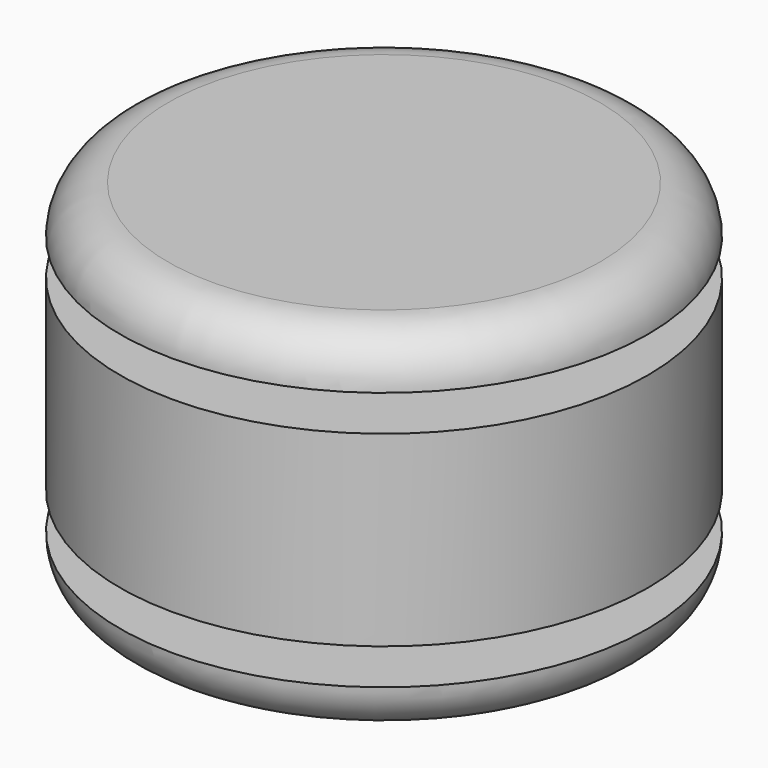
from build123d import *
from build123d import SkipClean  # not in build123d's __all__

# Parameters (mm, degrees)
F0_R      = 5.4
F1_DEPTH  = 1.5
F2_R      = 8.4
F2_R_2    = 6.4
F3_DEPTH  = 4.8
F4_R      = 11
F4_R_2    = 8.5
F5_DEPTH  = 7.8
F6_R      = 11
F6_R_2    = 5.4
F7_DEPTH  = 1.5
F8_R      = 3.15
F9_DEPTH  = 4.8
F10_R     = 4.15
F11_DEPTH = 3
F12_R     = 11
F13_DEPTH = 2
F14_R     = 1.9
F15_DEPTH = 7.4
F16_R     = 1.99999
F17_R     = 4.15
F18_DEPTH = 3
F19_R     = 11
F20_DEPTH = 2
F21_R     = 1.9
F22_DEPTH = 2.6
F23_R     = 1.99999


# Not quite as in the source:
# - a fillet or chamfer is up to 0.001 mm smaller than in the source, because OpenCascade refuses the exact size


with BuildPart() as f1:
    # F0 (on Top) → F1 (new body)
    with BuildSketch(Plane.XY):
        with BuildLine():
            ThreePointArc((2.5007633588, 8.0191135809), (0, 8.4), (-2.5007633588, 8.0191135809))
            ThreePointArc((-2.5007633588, 8.0191135809), (-7.2746133918, 4.2), (-8.1951377563, -1.8438321929))
            ThreePointArc((-8.1951377563, -1.8438321929), (-7.2746133918, -4.2), (-5.6943743975, -6.175281388))
            ThreePointArc((-5.6943743975, -6.175281388), (0, -8.4), (5.6943743975, -6.175281388))
            ThreePointArc((5.6943743975, -6.175281388), (7.2746133918, -4.2), (8.1951377563, -1.8438321929))
            ThreePointArc((8.1951377563, -1.8438321929), (7.2746133918, 4.2), (2.5007633588, 8.0191135809))
        make_face()
        Circle(F0_R, mode=Mode.SUBTRACT)
    extrude(amount=-F1_DEPTH)

    # F2 (on face) → F3 (join)
    with BuildSketch(Plane.XY):
        Circle(F2_R)
        Circle(F2_R_2, mode=Mode.SUBTRACT)
    with SkipClean():  # cleaning this boolean's faces spoils the solid; the shape is the same uncleaned
        extrude(amount=F3_DEPTH)


with BuildPart() as f5:
    # F4 (on face) → F5 (new body)
    with BuildSketch(Plane(origin=(0, 0, -1.5), x_dir=(1, 0, 0), z_dir=(0, 0, -1))):
        Circle(F4_R)
        Circle(F4_R_2, mode=Mode.SUBTRACT)
    extrude(amount=-F5_DEPTH)

    # F6 (on face) → F7 (join)
    with BuildSketch(Plane.XY.offset(6.3)):
        Circle(F6_R)
        Circle(F6_R_2, mode=Mode.SUBTRACT)
    extrude(amount=-F7_DEPTH)


with BuildPart() as f9:
    # F8 (on face) → F9 (new body)
    with BuildSketch(Plane.XY):
        Circle(F8_R)
    extrude(amount=F9_DEPTH)

    # F10 (on face) → F11 (join, through all)
    with BuildSketch(Plane(origin=(0, 0, 0), x_dir=(1, 0, 0), z_dir=(0, 0, -1))):
        Circle(F10_R)
    extrude(amount=F11_DEPTH)

    # F12 (on face) → F13 (join)
    with BuildSketch(Plane(origin=(0, 0, -3), x_dir=(1, 0, 0), z_dir=(0, 0, -1))):
        Circle(F12_R)
    extrude(amount=F13_DEPTH)

    # F14 (on face) → F15 (cut)
    with BuildSketch(Plane.XY.offset(4.8)):
        Circle(F14_R)
    extrude(amount=-F15_DEPTH, mode=Mode.SUBTRACT)

    # F16 (radius 2 in the source; OpenCascade refuses exactly that, so slightly less here)
    f16_edges = [f9.edges().sort_by_distance(p)[0] for p in [
        (-4.15, 0, -3),
        (-11, 0, -5),
    ]]
    fillet(f16_edges, radius=F16_R)


with BuildPart() as f18:
    # F17 (on face) → F18 (new body, through all)
    with BuildSketch(Plane.XY.offset(4.8)):
        Circle(F17_R)
    extrude(amount=F18_DEPTH)

    # F19 (on face) → F20 (join)
    with BuildSketch(Plane.XY.offset(7.8)):
        Circle(F19_R)
    extrude(amount=F20_DEPTH)

    # F21 (on face) → F22 (cut)
    with BuildSketch(Plane(origin=(0, 0, 4.8), x_dir=(1, 0, 0), z_dir=(0, 0, -1))):
        Circle(F21_R)
    extrude(amount=-F22_DEPTH, mode=Mode.SUBTRACT)

    # F23 (radius 2 in the source; OpenCascade refuses exactly that, so slightly less here)
    f23_edges = [f18.edges().sort_by_distance(p)[0] for p in [
        (-11, 0, 9.8),
        (-4.15, 0, 7.8),
    ]]
    fillet(f23_edges, radius=F23_R)


solid = Compound([f1.part, f5.part, f9.part, f18.part])
